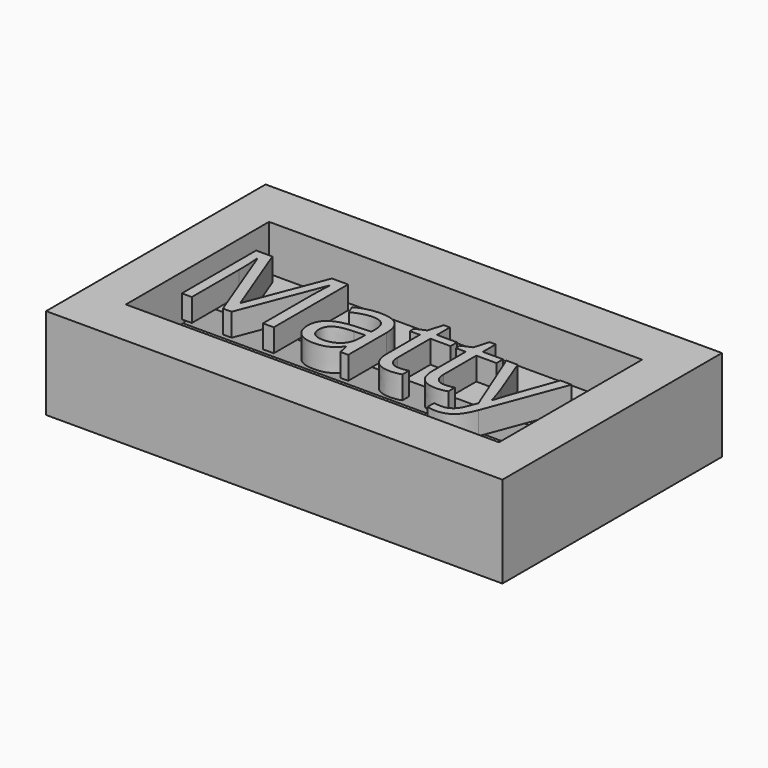
from build123d import *

# Parameters (mm, degrees)
F0_W         = 126.746
F0_H         = 76.2
F0_W_2       = 103.6245673895
F0_H_2       = 49.7092008591
F1_DEPTH     = 25.4
F2_DEPTH     = 12.7
F3_W         = 103.2421821728
F3_H         = 9.9418302998
F4_DEPTH     = 6.35
F5_TEXT_SIZE = 36.1135242403
F6_DEPTH     = 6.35


# Not quite as in the source:
# - Text() gives the source's letters only with a copy of the font that has no kerning and outlines rounded to 1/6400 em; it was checked with that copy


with BuildPart() as f1:
    # F0 (on Top) → F1 (new body)
    with BuildSketch(Plane.XY):
        Rectangle(F0_W, F0_H)
        Rectangle(F0_W_2, F0_H_2, mode=Mode.SUBTRACT)
    extrude(amount=F1_DEPTH)

    # F0 (on Top) → F2 (join)
    with BuildSketch(Plane.XY):
        Rectangle(F0_W_2, F0_H_2)
    extrude(amount=F2_DEPTH)

    # F3 (on face) → F4 (join)
    with BuildSketch(Plane.XY.offset(12.7)):
        with Locations((0.1911926083, 0)):
            Rectangle(F3_W, F3_H)
    extrude(amount=F4_DEPTH)

    # F5 (on face) → F6 (join)
    with BuildSketch(Plane.XY.offset(19.05)):
        with Locations((-49.1356253624, -13.1920538843)):
            Text('Matty', F5_TEXT_SIZE, font='Open Sans', text_align=(TextAlign.LEFT, TextAlign.BOTTOM))
    extrude(amount=F6_DEPTH)


solid = f1.part
